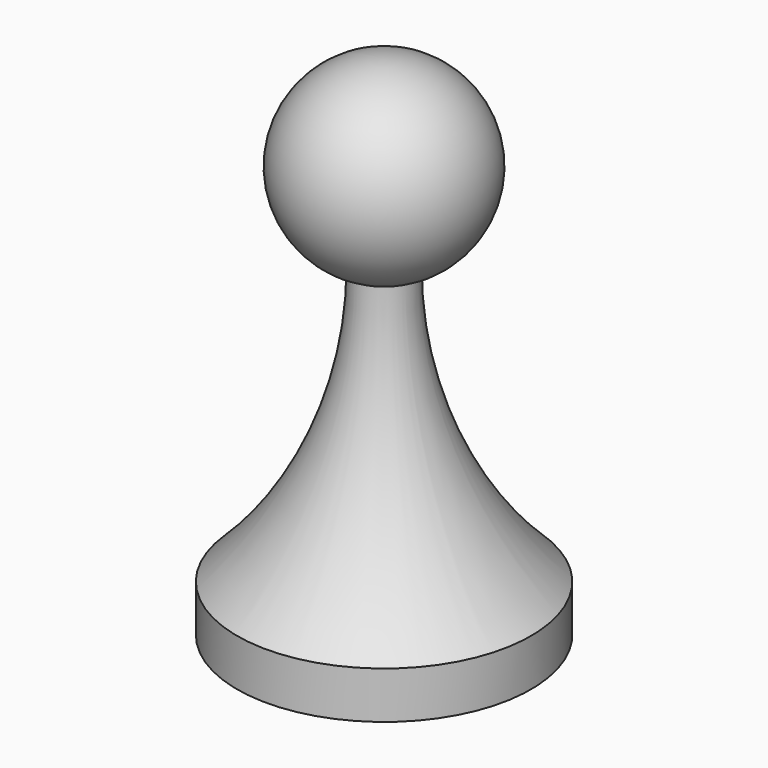
from build123d import *


# Not quite as in the source:
# - a feature of the source that left no trace in its solid (it failed there, or was rolled back) is left out


with BuildPart() as f1:
    # F0 (on Front) → F1 (revolve)
    with BuildSketch(Plane.XZ):
        with BuildLine():
            ThreePointArc((-2.5, 27.4883110198), (-1.2659509046, 27.1884526113), (0, 27.0876530966))
            Line((0, 27.0876530966), (0, 43.0876530966))
            ThreePointArc((0, 43.0876530966), (-7.8992004853, 36.3536040012), (-2.5, 27.4883110198))
        make_face()
    revolve(axis=Axis((0, 0, 35.0876530966), (0, 0, -1)))

    # F0 (on Front) → F2 (revolve)
    with BuildSketch(Plane.XZ):
        with BuildLine():
            ThreePointArc((-2.5, 27.4883110198), (-5.1040521689, 14.7240958602), (-12.5, 4))
            Line((-12.5, 4), (-2.5, 4))
            Line((-2.5, 4), (-2.5, 27.4883110198))
        make_face()
        with BuildLine():
            Line((-2.5, 4), (0, 4))
            Line((0, 4), (0, 27.0876530966))
            ThreePointArc((0, 27.0876530966), (-1.2659509046, 27.1884526113), (-2.5, 27.4883110198))
            Line((-2.5, 27.4883110198), (-2.5, 4))
        make_face()
    revolve(axis=Axis((0, 0, 15.5438265483), (0, 0, -1)))

    # F0 (on Front) → F3 (revolve)
    with BuildSketch(Plane.XZ):
        Polygon((-12.5, 0), (0, 0), (0, 4), (-2.5, 4), (-12.5, 4), align=None)
        with BuildLine():
            Line((-2.5, 4), (0, 4))
            Line((0, 4), (0, 27.0876530966))
            ThreePointArc((0, 27.0876530966), (-1.2659509046, 27.1884526113), (-2.5, 27.4883110198))
            Line((-2.5, 27.4883110198), (-2.5, 4))
        make_face()
    revolve(axis=Axis((0, 0, 2), (0, 0, 1)))


solid = f1.part
